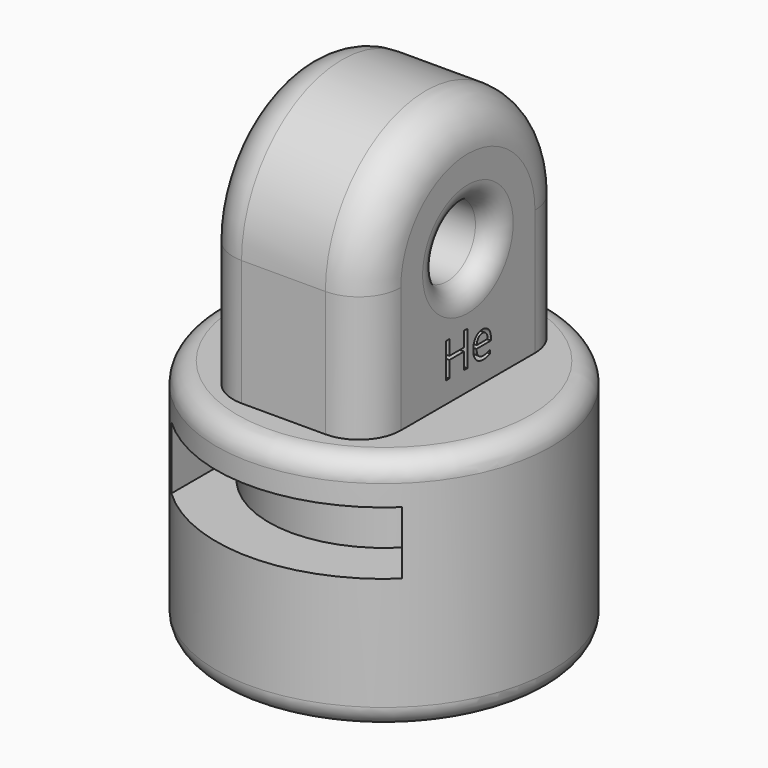
from build123d import *

# Parameters (mm, degrees)
F0_R          = 7
F1_DEPTH      = 9.4
F2_R          = 5.5
F3_DEPTH      = 8.9
F4_W          = 11
F4_H          = 10
F5_DEPTH      = 3
F6_R          = 7
F7_DEPTH      = 2
F8_R          = 1
F9_DEPTH      = 12.5
F10_R         = 1.7
F11_DEPTH     = 4
F12_R         = 1.2
F13_DEPTH     = 4.7968406421
F14_T1_DEPTH  = 6
F14_T4_ANGLE  = 180
F15_T1_DEPTH  = 6
F15_T4_ANGLE  = 180
F16_R         = 1
F17_R         = 0.5
F18_R         = 0.5
F19_TEXT_SIZE = 2.3244774241
F20_DEPTH     = 0.5
F21_R         = 8
F21_R_2       = 7
F22_DEPTH     = 11.4
F23_DEPTH     = 3
F24_DEPTH     = 12.5
F25_R         = 1
F26_R         = 1


# Not quite as in the source:
# - a fillet or chamfer that OpenCascade refuses, or shapes differently, is made with other operations: its cross-section is extruded or revolved along the edge and cut away or added
# - Text() gives the source's letters only with a copy of the font that has no kerning and outlines rounded to 1/6400 em; it was checked with that copy


with BuildPart() as f1:
    # F0 (on Top) → F1 (new body)
    with BuildSketch(Plane.XY):
        Circle(F0_R)
    extrude(amount=F1_DEPTH)

    # F2 (on face) → F3 (cut)
    with BuildSketch(Plane.XY.offset(9.4)):
        Circle(F2_R)
    extrude(amount=-F3_DEPTH, mode=Mode.SUBTRACT)

    # F4 (on face) → F5 (cut)
    with BuildSketch(Plane.XY.offset(9.4)):
        with Locations((0, -5)):
            Rectangle(F4_W, F4_H)
    extrude(amount=-F5_DEPTH, mode=Mode.SUBTRACT)

    # F6 (on face) → F7 (join)
    with BuildSketch(Plane.XY.offset(9.4)):
        Circle(F6_R)
    extrude(amount=F7_DEPTH)

    # F8 (on Front) → F9 (cut, symmetric)
    with BuildSketch(Plane.XZ):
        with Locations((0, 7.9)):
            Circle(F8_R)
    extrude(amount=F9_DEPTH, both=True, mode=Mode.SUBTRACT)

    # F10 (on Right) → F11 (join, symmetric)
    with BuildSketch(Plane.YZ):
        with BuildLine():
            Line((-6, 11.4), (6, 11.4))
            Line((6, 11.4), (6, 17.4))
            ThreePointArc((6, 17.4), (0, 23.4), (-6, 17.4))
            Line((-6, 17.4), (-6, 11.4))
        make_face()
        with Locations((0, 17.4)):
            Circle(F10_R, mode=Mode.SUBTRACT)
    extrude(amount=F11_DEPTH, both=True)

    # F12 (on face) → F13 (cut, through all)
    with BuildSketch(Plane(origin=(0, 6, 0), x_dir=(-1, 0, 0), z_dir=(0, 1, 0))):
        with Locations((0, 17.4)):
            Circle(F12_R)
    extrude(amount=-F13_DEPTH, mode=Mode.SUBTRACT)

    # F14: fillet of radius 2 on 3 edges, made by hand

    # F14_s2 → F14_t1 (cut)
    with BuildSketch(Plane.XY.offset(11.4)):
        with BuildLine():
            ThreePointArc((4, 4), (3.4142135624, 5.4142135624), (2, 6))
            Line((2, 6), (4, 6))
            Line((4, 6), (4, 4))
        make_face()
        with BuildLine():
            ThreePointArc((4, -4), (3.4142135624, -5.4142135624), (2, -6))
            Line((2, -6), (4, -6))
            Line((4, -6), (4, -4))
        make_face()
    extrude(amount=F14_T1_DEPTH, mode=Mode.SUBTRACT)

    # F14_s3 → F14_t4 (revolve, cut)
    with BuildSketch(Plane.XY.offset(17.4)):
        with BuildLine():
            ThreePointArc((4, 4), (3.4142135624, 5.4142135624), (2, 6))
            Line((2, 6), (4, 6))
            Line((4, 6), (4, 4))
        make_face()
    revolve(axis=Axis((4, 0, 17.4), (1, 0, 0)), revolution_arc=F14_T4_ANGLE, mode=Mode.SUBTRACT)

    # F15: fillet of radius 2 on 3 edges, made by hand

    # F15_s2 → F15_t1 (cut)
    with BuildSketch(Plane.XY.offset(11.4)):
        with BuildLine():
            ThreePointArc((-2, 6), (-3.4142135624, 5.4142135624), (-4, 4))
            Line((-4, 4), (-4, 6))
            Line((-4, 6), (-2, 6))
        make_face()
        with BuildLine():
            ThreePointArc((-2, -6), (-3.4142135624, -5.4142135624), (-4, -4))
            Line((-4, -4), (-4, -6))
            Line((-4, -6), (-2, -6))
        make_face()
    extrude(amount=F15_T1_DEPTH, mode=Mode.SUBTRACT)

    # F15_s3 → F15_t4 (revolve, cut)
    with BuildSketch(Plane.XY.offset(17.4)):
        with BuildLine():
            ThreePointArc((-4, 4), (-3.4142135624, 5.4142135624), (-2, 6))
            Line((-2, 6), (-4, 6))
            Line((-4, 6), (-4, 4))
        make_face()
    revolve(axis=Axis((-4, 0, 17.4), (1, 0, 0)), revolution_arc=F15_T4_ANGLE, mode=Mode.SUBTRACT)

    # F16
    f16_edges = [f1.edges().sort_by_distance(p)[0] for p in [
        (-4, -1.7, 17.4),
        (4, -1.7, 17.4),
    ]]
    fillet(f16_edges, radius=F16_R)

    # F17
    f17_edges = [f1.edges().sort_by_distance(p)[0] for p in [
        (-1, 6.928203, 7.9),
    ]]
    fillet(f17_edges, radius=F17_R)

    # F18
    f18_edges = [f1.edges().sort_by_distance(p)[0] for p in [
        (0, 5.878775, 18.6),
        (0, 6, 16.2),
    ]]
    fillet(f18_edges, radius=F18_R)

    # F19 (on face) → F20 (cut)
    with BuildSketch(Plane.YZ.offset(4)):
        with Locations((-1.524167111, 12.4)):
            Text('He', F19_TEXT_SIZE, font='Open Sans', text_align=(TextAlign.LEFT, TextAlign.BOTTOM))
    extrude(amount=-F20_DEPTH, mode=Mode.SUBTRACT)

    # F21 (on Top) → F22 (join)
    with BuildSketch(Plane.XY):
        Circle(F21_R)
        Circle(F21_R_2, mode=Mode.SUBTRACT)
    extrude(amount=F22_DEPTH)

    # F4 (on face) → F23 (cut)
    with BuildSketch(Plane.XY.offset(9.4)):
        with Locations((0, -5)):
            Rectangle(F4_W, F4_H)
    extrude(amount=-F23_DEPTH, mode=Mode.SUBTRACT)

    # F8 (on Front) → F24 (cut, symmetric)
    with BuildSketch(Plane.XZ):
        with Locations((0, 7.9)):
            Circle(F8_R)
    extrude(amount=F24_DEPTH, both=True, mode=Mode.SUBTRACT)

    # F25
    f25_edges = [f1.edges().sort_by_distance(p)[0] for p in [
        (-8, 0, 11.4),
    ]]
    fillet(f25_edges, radius=F25_R)

    # F26
    f26_edges = [f1.edges().sort_by_distance(p)[0] for p in [
        (-8, 0, 0),
    ]]
    fillet(f26_edges, radius=F26_R)


solid = f1.part
